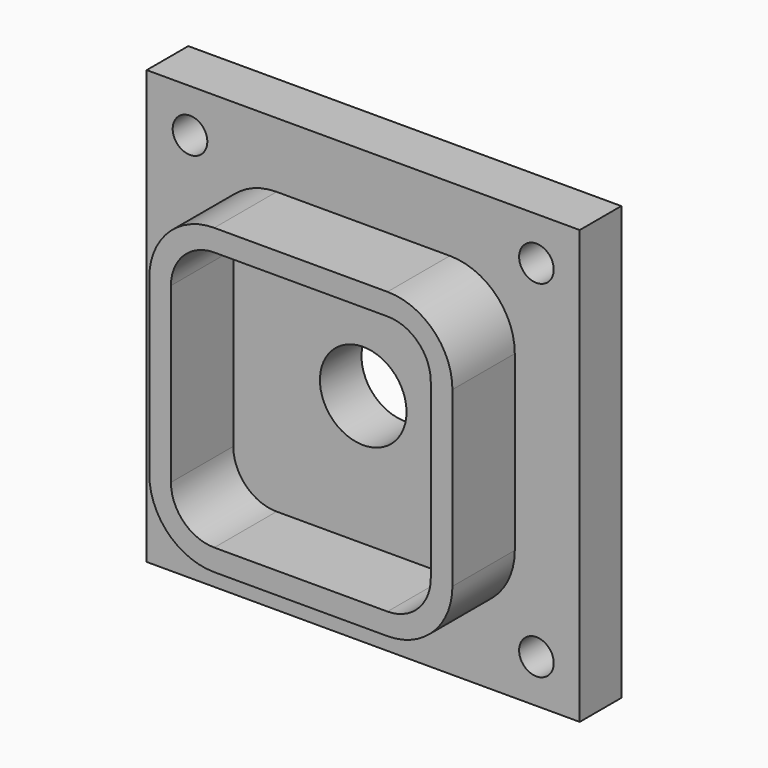
from build123d import *

# Parameters (mm, degrees)
F0_W     = 100
F0_H     = 100
F0_R     = 4
F0_R_2   = 10
F1_DEPTH = 12
F2_DEPTH = 30
F3_DEPTH = 25


with BuildPart() as f1:
    # F0 (on Front) → F1 (new body)
    with BuildSketch(Plane.XZ):
        Rectangle(F0_W, F0_H)
        with Locations((-40, -40)):
            Circle(F0_R, mode=Mode.SUBTRACT)
        with Locations((40, -40)):
            Circle(F0_R, mode=Mode.SUBTRACT)
        with Locations((-40, 40)):
            Circle(F0_R, mode=Mode.SUBTRACT)
        with BuildLine():
            Line((-35, -20), (-35, 0))
            Line((-35, 0), (-35, 20))
            ThreePointArc((-35, 20), (-30.6066017178, 30.6066017178), (-20, 35))
            Line((-20, 35), (0, 35))
            Line((0, 35), (20, 35))
            ThreePointArc((20, 35), (30.6066017178, 30.6066017178), (35, 20))
            Line((35, 20), (35, 0))
            Line((35, 0), (35, -20))
            ThreePointArc((35, -20), (30.6066017178, -30.6066017178), (20, -35))
            Line((20, -35), (0, -35))
            Line((0, -35), (-20, -35))
            ThreePointArc((-20, -35), (-30.6066017178, -30.6066017178), (-35, -20))
        make_face(mode=Mode.SUBTRACT)
        with Locations((40, 40)):
            Circle(F0_R, mode=Mode.SUBTRACT)
        with BuildLine():
            Line((-35, 20), (-35, 0))
            Line((-35, 0), (-35, -20))
            ThreePointArc((-35, -20), (-30.6066017178, -30.6066017178), (-20, -35))
            Line((-20, -35), (0, -35))
            Line((0, -35), (20, -35))
            ThreePointArc((20, -35), (30.6066017178, -30.6066017178), (35, -20))
            Line((35, -20), (35, 0))
            Line((35, 0), (35, 20))
            ThreePointArc((35, 20), (30.6066017178, 30.6066017178), (20, 35))
            Line((20, 35), (0, 35))
            Line((0, 35), (-20, 35))
            ThreePointArc((-20, 35), (-30.6066017178, 30.6066017178), (-35, 20))
        make_face()
        with BuildLine():
            Line((-30, -20), (-30, 0))
            Line((-30, 0), (-30, 20))
            ThreePointArc((-30, 20), (-27.0710678119, 27.0710678119), (-20, 30))
            Line((-20, 30), (0, 30))
            Line((0, 30), (20, 30))
            ThreePointArc((20, 30), (27.0710678119, 27.0710678119), (30, 20))
            Line((30, 20), (30, 0))
            Line((30, 0), (30, -20))
            ThreePointArc((30, -20), (27.0710678119, -27.0710678119), (20, -30))
            Line((20, -30), (0, -30))
            Line((0, -30), (-20, -30))
            ThreePointArc((-20, -30), (-27.0710678119, -27.0710678119), (-30, -20))
        make_face(mode=Mode.SUBTRACT)
        with BuildLine():
            Line((-30, 20), (-30, 0))
            Line((-30, 0), (-30, -20))
            ThreePointArc((-30, -20), (-27.0710678119, -27.0710678119), (-20, -30))
            Line((-20, -30), (0, -30))
            Line((0, -30), (20, -30))
            ThreePointArc((20, -30), (27.0710678119, -27.0710678119), (30, -20))
            Line((30, -20), (30, 0))
            Line((30, 0), (30, 20))
            ThreePointArc((30, 20), (27.0710678119, 27.0710678119), (20, 30))
            Line((20, 30), (0, 30))
            Line((0, 30), (-20, 30))
            ThreePointArc((-20, 30), (-27.0710678119, 27.0710678119), (-30, 20))
        make_face()
        Circle(F0_R_2, mode=Mode.SUBTRACT)
    extrude(amount=F1_DEPTH)

    # F0 (on Front) → F2 (join)
    with BuildSketch(Plane.XZ):
        with BuildLine():
            Line((-35, 20), (-35, 0))
            Line((-35, 0), (-35, -20))
            ThreePointArc((-35, -20), (-30.6066017178, -30.6066017178), (-20, -35))
            Line((-20, -35), (0, -35))
            Line((0, -35), (20, -35))
            ThreePointArc((20, -35), (30.6066017178, -30.6066017178), (35, -20))
            Line((35, -20), (35, 0))
            Line((35, 0), (35, 20))
            ThreePointArc((35, 20), (30.6066017178, 30.6066017178), (20, 35))
            Line((20, 35), (0, 35))
            Line((0, 35), (-20, 35))
            ThreePointArc((-20, 35), (-30.6066017178, 30.6066017178), (-35, 20))
        make_face()
        with BuildLine():
            Line((-30, -20), (-30, 0))
            Line((-30, 0), (-30, 20))
            ThreePointArc((-30, 20), (-27.0710678119, 27.0710678119), (-20, 30))
            Line((-20, 30), (0, 30))
            Line((0, 30), (20, 30))
            ThreePointArc((20, 30), (27.0710678119, 27.0710678119), (30, 20))
            Line((30, 20), (30, 0))
            Line((30, 0), (30, -20))
            ThreePointArc((30, -20), (27.0710678119, -27.0710678119), (20, -30))
            Line((20, -30), (0, -30))
            Line((0, -30), (-20, -30))
            ThreePointArc((-20, -30), (-27.0710678119, -27.0710678119), (-30, -20))
        make_face(mode=Mode.SUBTRACT)
    extrude(amount=F2_DEPTH)

    # F0 (on Front) → F3 (cut)
    with BuildSketch(Plane.XZ):
        with Locations((-40, 40)):
            Circle(F0_R)
        with Locations((40, 40)):
            Circle(F0_R)
        with Locations((-40, -40)):
            Circle(F0_R)
        with Locations((40, -40)):
            Circle(F0_R)
    extrude(amount=-F3_DEPTH, mode=Mode.SUBTRACT)


solid = f1.part
